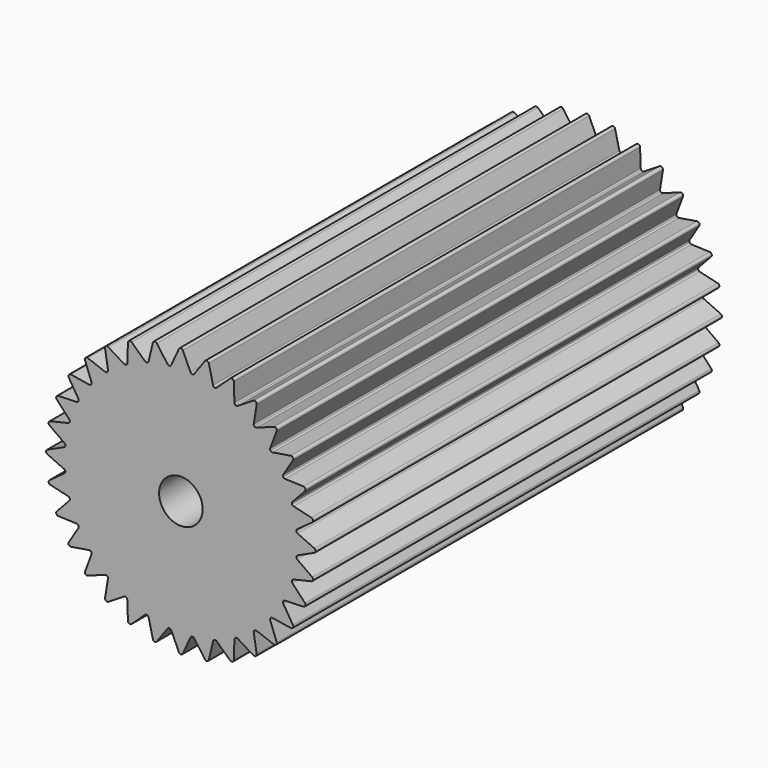
from build123d import *

# Parameters (mm, degrees)
F0_R            = 8
F0_R_2          = 5
F1_DEPTH        = 35
F2_DEPTH        = 20
F5_DEPTH        = 35
F5_COPIES_COUNT = 32
F6_T1_DEPTH     = 35
F6_T3_DEPTH     = 36.6415271023
F7_R            = 1.5
F8_DEPTH        = 8
F9_R            = 6
F10_DEPTH       = 25


# Not quite as in the source:
# - a fillet or chamfer that OpenCascade refuses, or shapes differently, is made with other operations: its cross-section is extruded or revolved along the edge and cut away or added
# - a pattern or mirror of a feature is missing from the dataset's text; its kind, count and spacing are read off the source's solid


with BuildPart() as f1:
    # F0 (on Front) → F1 (new body)
    with BuildSketch(Plane.XZ):
        Circle(F0_R)
        Circle(F0_R_2, mode=Mode.SUBTRACT)
        Circle(F0_R_2)
    extrude(amount=F1_DEPTH)

    # F0 (on Front) → F2 (join)
    with BuildSketch(Plane.XZ):
        Circle(F0_R_2)
    extrude(amount=F2_DEPTH)

    # F4 (on face) → F5 (join)
    with BuildSketch(Plane(origin=(0, 0, 0), x_dir=(-1, 0, 0), z_dir=(0, 1, 0))):
        with BuildLine():
            ThreePointArc((-0.6993297572, 7.969375), (-0.35, 7.9923400829), (0, 8))
            ThreePointArc((0, 8), (0.35, 7.9923400829), (0.6993297572, 7.969375))
            Line((0.6993297572, 7.969375), (0, 9.5))
            Line((0, 9.5), (-0.6993297572, 7.969375))
        make_face()
    f5 = extrude(amount=-F5_DEPTH)

    # F5_copies: F5 ×32 about axis
    f5_copies_axis = Axis((0, 0, 0), (0, 1, 0))
    for i in range(1, F5_COPIES_COUNT):
        add(f5.rotate(f5_copies_axis, i * 360 / F5_COPIES_COUNT))

    # F6: fillet of radius 0.15 on 96 edges, made by hand

    # F6_s2 → F6_t1 (join)
    with BuildSketch(Plane.XZ):
        with BuildLine():
            ThreePointArc((0.6632529517, 8.0483364054), (0.7125009612, 7.9886122754), (0.7849689133, 7.9613958453))
            ThreePointArc((0.7849689133, 7.9613958453), (0.7421600586, 7.9655005146), (0.6993297572, 7.969375))
            Line((0.6993297572, 7.969375), (0.6632529517, 8.0483364054))
        make_face()
        with BuildLine():
            ThreePointArc((-0.7849689133, 7.9613958453), (-0.7125009612, 7.9886122754), (-0.6632529517, 8.0483364054))
            Line((-0.6632529517, 8.0483364054), (-0.6993297572, 7.969375))
            ThreePointArc((-0.6993297572, 7.969375), (-0.7421600586, 7.9655005146), (-0.7849689133, 7.9613958453))
        make_face()
        with BuildLine():
            ThreePointArc((-0.7833053234, 7.9615596946), (-0.8596904862, 7.9741153725), (-0.9196438088, 8.0230841101))
            Line((-0.9196438088, 8.0230841101), (-0.868855603, 7.9526781616))
            ThreePointArc((-0.868855603, 7.9526781616), (-0.8260923992, 7.9572339005), (-0.7833053234, 7.9615596946))
        make_face()
        with BuildLine():
            ThreePointArc((-2.3214775758, 7.6557652697), (-2.3988445104, 7.6531776878), (-2.4671991735, 7.6895091918))
            Line((-2.4671991735, 7.6895091918), (-2.4036513296, 7.6303643613))
            ThreePointArc((-2.4036513296, 7.6303643613), (-2.3625985894, 7.6431752502), (-2.3214775758, 7.6557652697))
        make_face()
        with BuildLine():
            ThreePointArc((-2.3230772349, 7.6552800184), (-2.2573113963, 7.6961112886), (-2.2206612733, 7.7642956462))
            Line((-2.2206612733, 7.7642956462), (-2.2406402671, 7.6798132265))
            ThreePointArc((-2.2406402671, 7.6798132265), (-2.2818917216, 7.6676574109), (-2.3230772349, 7.6552800184))
        make_face()
        with BuildLine():
            ThreePointArc((-3.6927308274, 7.1818773596), (-3.7153746204, 7.107853061), (-3.7719110012, 7.0549760736))
            ThreePointArc((-3.7719110012, 7.0549760736), (-3.7339315654, 7.075150533), (-3.695844228, 7.0951205375))
            Line((-3.695844228, 7.0951205375), (-3.6927308274, 7.1818773596))
        make_face()
        with BuildLine():
            ThreePointArc((-3.7704367469, 7.0557640789), (-3.8458122853, 7.0381326765), (-3.9199414575, 7.0604307476))
            Line((-3.9199414575, 7.0604307476), (-3.8460760836, 7.0148199377))
            ThreePointArc((-3.8460760836, 7.0148199377), (-3.8083114408, 7.0353936613), (-3.7704367469, 7.0557640789))
        make_face()
        with BuildLine():
            ThreePointArc((-5.0228908068, 6.3234635537), (-5.0306580813, 6.2464440264), (-5.0757923429, 6.1835533548))
            ThreePointArc((-5.0757923429, 6.1835533548), (-5.0424785132, 6.2107495879), (-5.0090189679, 6.2377663454))
            Line((-5.0090189679, 6.2377663454), (-5.0228908068, 6.3234635537))
        make_face()
        with BuildLine():
            ThreePointArc((-5.0745001483, 6.1846138315), (-5.1449876509, 6.1526161735), (-5.2220425897, 6.1600239093))
            Line((-5.2220425897, 6.1600239093), (-5.1406982907, 6.129699918))
            ThreePointArc((-5.1406982907, 6.129699918), (-5.1076730192, 6.1572458396), (-5.0745001483, 6.1846138315))
        make_face()
        with BuildLine():
            ThreePointArc((-6.1600239093, 5.2220425897), (-6.1526161735, 5.1449876509), (-6.1846138315, 5.0745001483))
            ThreePointArc((-6.1846138315, 5.0745001483), (-6.1572458396, 5.1076730192), (-6.129699918, 5.1406982907))
            Line((-6.129699918, 5.1406982907), (-6.1600239093, 5.2220425897))
        make_face()
        with BuildLine():
            ThreePointArc((-6.1835533548, 5.0757923429), (-6.2464440264, 5.0306580813), (-6.3234635537, 5.0228908068))
            Line((-6.3234635537, 5.0228908068), (-6.2377663454, 5.0090189679))
            ThreePointArc((-6.2377663454, 5.0090189679), (-6.2107495879, 5.0424785132), (-6.1835533548, 5.0757923429))
        make_face()
        with BuildLine():
            ThreePointArc((-7.0604307476, 3.9199414575), (-7.0381326765, 3.8458122853), (-7.0557640789, 3.7704367469))
            ThreePointArc((-7.0557640789, 3.7704367469), (-7.0353936613, 3.8083114408), (-7.0148199377, 3.8460760836))
            Line((-7.0148199377, 3.8460760836), (-7.0604307476, 3.9199414575))
        make_face()
        with BuildLine():
            ThreePointArc((-7.0549760736, 3.7719110012), (-7.107853061, 3.7153746204), (-7.1818773596, 3.6927308274))
            Line((-7.1818773596, 3.6927308274), (-7.0951205375, 3.695844228))
            ThreePointArc((-7.0951205375, 3.695844228), (-7.075150533, 3.7339315654), (-7.0549760736, 3.7719110012))
        make_face()
        with BuildLine():
            ThreePointArc((-7.6895091918, 2.4671991735), (-7.6531776878, 2.3988445104), (-7.6557652697, 2.3214775758))
            ThreePointArc((-7.6557652697, 2.3214775758), (-7.6431752502, 2.3625985894), (-7.6303643613, 2.4036513296))
            Line((-7.6303643613, 2.4036513296), (-7.6895091918, 2.4671991735))
        make_face()
        with BuildLine():
            ThreePointArc((-7.6552800184, 2.3230772349), (-7.6961112886, 2.2573113963), (-7.7642956462, 2.2206612733))
            Line((-7.7642956462, 2.2206612733), (-7.6798132265, 2.2406402671))
            ThreePointArc((-7.6798132265, 2.2406402671), (-7.6676574109, 2.2818917216), (-7.6552800184, 2.3230772349))
        make_face()
        with BuildLine():
            ThreePointArc((-8.0230841101, 0.9196438088), (-7.9741153725, 0.8596904862), (-7.9615596946, 0.7833053234))
            ThreePointArc((-7.9615596946, 0.7833053234), (-7.9572339005, 0.8260923992), (-7.9526781616, 0.868855603))
            Line((-7.9526781616, 0.868855603), (-8.0230841101, 0.9196438088))
        make_face()
        with BuildLine():
            ThreePointArc((-7.9613958453, 0.7849689133), (-7.9886122754, 0.7125009612), (-8.0483364054, 0.6632529517))
            Line((-8.0483364054, 0.6632529517), (-7.969375, 0.6993297572))
            ThreePointArc((-7.969375, 0.6993297572), (-7.9655005146, 0.7421600586), (-7.9613958453, 0.7849689133))
        make_face()
        with BuildLine():
            ThreePointArc((-8.0483364054, -0.6632529517), (-7.9886122754, -0.7125009612), (-7.9613958453, -0.7849689133))
            ThreePointArc((-7.9613958453, -0.7849689133), (-7.9655005146, -0.7421600586), (-7.969375, -0.6993297572))
            Line((-7.969375, -0.6993297572), (-8.0483364054, -0.6632529517))
        make_face()
        with BuildLine():
            ThreePointArc((-7.9615596946, -0.7833053234), (-7.9741153725, -0.8596904862), (-8.0230841101, -0.9196438088))
            Line((-8.0230841101, -0.9196438088), (-7.9526781616, -0.868855603))
            ThreePointArc((-7.9526781616, -0.868855603), (-7.9572339005, -0.8260923992), (-7.9615596946, -0.7833053234))
        make_face()
        with BuildLine():
            ThreePointArc((-7.7642956462, -2.2206612733), (-7.6961112886, -2.2573113963), (-7.6552800184, -2.3230772349))
            ThreePointArc((-7.6552800184, -2.3230772349), (-7.6676574109, -2.2818917216), (-7.6798132265, -2.2406402671))
            Line((-7.6798132265, -2.2406402671), (-7.7642956462, -2.2206612733))
        make_face()
        with BuildLine():
            ThreePointArc((-7.6557652697, -2.3214775758), (-7.6531776878, -2.3988445104), (-7.6895091918, -2.4671991735))
            Line((-7.6895091918, -2.4671991735), (-7.6303643613, -2.4036513296))
            ThreePointArc((-7.6303643613, -2.4036513296), (-7.6431752502, -2.3625985894), (-7.6557652697, -2.3214775758))
        make_face()
        with BuildLine():
            ThreePointArc((-7.1818773596, -3.6927308274), (-7.107853061, -3.7153746204), (-7.0549760736, -3.7719110012))
            ThreePointArc((-7.0549760736, -3.7719110012), (-7.075150533, -3.7339315654), (-7.0951205375, -3.695844228))
            Line((-7.0951205375, -3.695844228), (-7.1818773596, -3.6927308274))
        make_face()
        with BuildLine():
            ThreePointArc((-7.0557640789, -3.7704367469), (-7.0381326765, -3.8458122853), (-7.0604307476, -3.9199414575))
            Line((-7.0604307476, -3.9199414575), (-7.0148199377, -3.8460760836))
            ThreePointArc((-7.0148199377, -3.8460760836), (-7.0353936613, -3.8083114408), (-7.0557640789, -3.7704367469))
        make_face()
        with BuildLine():
            ThreePointArc((-6.3234635537, -5.0228908068), (-6.2464440264, -5.0306580813), (-6.1835533548, -5.0757923429))
            ThreePointArc((-6.1835533548, -5.0757923429), (-6.2107495879, -5.0424785132), (-6.2377663454, -5.0090189679))
            Line((-6.2377663454, -5.0090189679), (-6.3234635537, -5.0228908068))
        make_face()
        with BuildLine():
            ThreePointArc((-6.1846138315, -5.0745001483), (-6.1526161735, -5.1449876509), (-6.1600239093, -5.2220425897))
            Line((-6.1600239093, -5.2220425897), (-6.129699918, -5.1406982907))
            ThreePointArc((-6.129699918, -5.1406982907), (-6.1572458396, -5.1076730192), (-6.1846138315, -5.0745001483))
        make_face()
        with BuildLine():
            ThreePointArc((-5.2220425897, -6.1600239093), (-5.1449876509, -6.1526161735), (-5.0745001483, -6.1846138315))
            ThreePointArc((-5.0745001483, -6.1846138315), (-5.1076730192, -6.1572458396), (-5.1406982907, -6.129699918))
            Line((-5.1406982907, -6.129699918), (-5.2220425897, -6.1600239093))
        make_face()
        with BuildLine():
            ThreePointArc((-5.0757923429, -6.1835533548), (-5.0306580813, -6.2464440264), (-5.0228908068, -6.3234635537))
            Line((-5.0228908068, -6.3234635537), (-5.0090189679, -6.2377663454))
            ThreePointArc((-5.0090189679, -6.2377663454), (-5.0424785132, -6.2107495879), (-5.0757923429, -6.1835533548))
        make_face()
        with BuildLine():
            ThreePointArc((-3.9199414575, -7.0604307476), (-3.8458122853, -7.0381326765), (-3.7704367469, -7.0557640789))
            ThreePointArc((-3.7704367469, -7.0557640789), (-3.8083114408, -7.0353936613), (-3.8460760836, -7.0148199377))
            Line((-3.8460760836, -7.0148199377), (-3.9199414575, -7.0604307476))
        make_face()
        with BuildLine():
            ThreePointArc((-3.7719110012, -7.0549760736), (-3.7153746204, -7.107853061), (-3.6927308274, -7.1818773596))
            Line((-3.6927308274, -7.1818773596), (-3.695844228, -7.0951205375))
            ThreePointArc((-3.695844228, -7.0951205375), (-3.7339315654, -7.075150533), (-3.7719110012, -7.0549760736))
        make_face()
        with BuildLine():
            ThreePointArc((-2.4671991735, -7.6895091918), (-2.3988445104, -7.6531776878), (-2.3214775758, -7.6557652697))
            ThreePointArc((-2.3214775758, -7.6557652697), (-2.3625985894, -7.6431752502), (-2.4036513296, -7.6303643613))
            Line((-2.4036513296, -7.6303643613), (-2.4671991735, -7.6895091918))
        make_face()
        with BuildLine():
            ThreePointArc((-2.3230772349, -7.6552800184), (-2.2573113963, -7.6961112886), (-2.2206612733, -7.7642956462))
            Line((-2.2206612733, -7.7642956462), (-2.2406402671, -7.6798132265))
            ThreePointArc((-2.2406402671, -7.6798132265), (-2.2818917216, -7.6676574109), (-2.3230772349, -7.6552800184))
        make_face()
        with BuildLine():
            ThreePointArc((-0.9196438088, -8.0230841101), (-0.8596904862, -7.9741153725), (-0.7833053234, -7.9615596946))
            ThreePointArc((-0.7833053234, -7.9615596946), (-0.8260923992, -7.9572339005), (-0.868855603, -7.9526781616))
            Line((-0.868855603, -7.9526781616), (-0.9196438088, -8.0230841101))
        make_face()
        with BuildLine():
            ThreePointArc((-0.7849689133, -7.9613958453), (-0.7125009612, -7.9886122754), (-0.6632529517, -8.0483364054))
            Line((-0.6632529517, -8.0483364054), (-0.6993297572, -7.969375))
            ThreePointArc((-0.6993297572, -7.969375), (-0.7421600586, -7.9655005146), (-0.7849689133, -7.9613958453))
        make_face()
        with BuildLine():
            ThreePointArc((0.6632529517, -8.0483364054), (0.7125009612, -7.9886122754), (0.7849689133, -7.9613958453))
            ThreePointArc((0.7849689133, -7.9613958453), (0.7421600586, -7.9655005146), (0.6993297572, -7.969375))
            Line((0.6993297572, -7.969375), (0.6632529517, -8.0483364054))
        make_face()
        with BuildLine():
            ThreePointArc((0.7833053234, -7.9615596946), (0.8596904862, -7.9741153725), (0.9196438088, -8.0230841101))
            Line((0.9196438088, -8.0230841101), (0.868855603, -7.9526781616))
            ThreePointArc((0.868855603, -7.9526781616), (0.8260923992, -7.9572339005), (0.7833053234, -7.9615596946))
        make_face()
        with BuildLine():
            ThreePointArc((2.2206612733, -7.7642956462), (2.2573113963, -7.6961112886), (2.3230772349, -7.6552800184))
            ThreePointArc((2.3230772349, -7.6552800184), (2.2818917216, -7.6676574109), (2.2406402671, -7.6798132265))
            Line((2.2406402671, -7.6798132265), (2.2206612733, -7.7642956462))
        make_face()
        with BuildLine():
            ThreePointArc((2.3214775758, -7.6557652697), (2.3988445104, -7.6531776878), (2.4671991735, -7.6895091918))
            Line((2.4671991735, -7.6895091918), (2.4036513296, -7.6303643613))
            ThreePointArc((2.4036513296, -7.6303643613), (2.3625985894, -7.6431752502), (2.3214775758, -7.6557652697))
        make_face()
        with BuildLine():
            ThreePointArc((3.6927308274, -7.1818773596), (3.7153746204, -7.107853061), (3.7719110012, -7.0549760736))
            ThreePointArc((3.7719110012, -7.0549760736), (3.7339315654, -7.075150533), (3.695844228, -7.0951205375))
            Line((3.695844228, -7.0951205375), (3.6927308274, -7.1818773596))
        make_face()
        with BuildLine():
            ThreePointArc((3.7704367469, -7.0557640789), (3.8458122853, -7.0381326765), (3.9199414575, -7.0604307476))
            Line((3.9199414575, -7.0604307476), (3.8460760836, -7.0148199377))
            ThreePointArc((3.8460760836, -7.0148199377), (3.8083114408, -7.0353936613), (3.7704367469, -7.0557640789))
        make_face()
        with BuildLine():
            ThreePointArc((5.0228908068, -6.3234635537), (5.0306580813, -6.2464440264), (5.0757923429, -6.1835533548))
            ThreePointArc((5.0757923429, -6.1835533548), (5.0424785132, -6.2107495879), (5.0090189679, -6.2377663454))
            Line((5.0090189679, -6.2377663454), (5.0228908068, -6.3234635537))
        make_face()
        with BuildLine():
            ThreePointArc((5.0745001483, -6.1846138315), (5.1449876509, -6.1526161735), (5.2220425897, -6.1600239093))
            Line((5.2220425897, -6.1600239093), (5.1406982907, -6.129699918))
            ThreePointArc((5.1406982907, -6.129699918), (5.1076730192, -6.1572458396), (5.0745001483, -6.1846138315))
        make_face()
        with BuildLine():
            ThreePointArc((6.1600239093, -5.2220425897), (6.1526161735, -5.1449876509), (6.1846138315, -5.0745001483))
            ThreePointArc((6.1846138315, -5.0745001483), (6.1572458396, -5.1076730192), (6.129699918, -5.1406982907))
            Line((6.129699918, -5.1406982907), (6.1600239093, -5.2220425897))
        make_face()
        with BuildLine():
            ThreePointArc((6.1835533548, -5.0757923429), (6.2464440264, -5.0306580813), (6.3234635537, -5.0228908068))
            Line((6.3234635537, -5.0228908068), (6.2377663454, -5.0090189679))
            ThreePointArc((6.2377663454, -5.0090189679), (6.2107495879, -5.0424785132), (6.1835533548, -5.0757923429))
        make_face()
        with BuildLine():
            ThreePointArc((7.0604307476, -3.9199414575), (7.0381326765, -3.8458122853), (7.0557640789, -3.7704367469))
            ThreePointArc((7.0557640789, -3.7704367469), (7.0353936613, -3.8083114408), (7.0148199377, -3.8460760836))
            Line((7.0148199377, -3.8460760836), (7.0604307476, -3.9199414575))
        make_face()
        with BuildLine():
            ThreePointArc((7.0549760736, -3.7719110012), (7.107853061, -3.7153746204), (7.1818773596, -3.6927308274))
            Line((7.1818773596, -3.6927308274), (7.0951205375, -3.695844228))
            ThreePointArc((7.0951205375, -3.695844228), (7.075150533, -3.7339315654), (7.0549760736, -3.7719110012))
        make_face()
        with BuildLine():
            ThreePointArc((7.6895091918, -2.4671991735), (7.6531776878, -2.3988445104), (7.6557652697, -2.3214775758))
            ThreePointArc((7.6557652697, -2.3214775758), (7.6431752502, -2.3625985894), (7.6303643613, -2.4036513296))
            Line((7.6303643613, -2.4036513296), (7.6895091918, -2.4671991735))
        make_face()
        with BuildLine():
            ThreePointArc((7.6552800184, -2.3230772349), (7.6961112886, -2.2573113963), (7.7642956462, -2.2206612733))
            Line((7.7642956462, -2.2206612733), (7.6798132265, -2.2406402671))
            ThreePointArc((7.6798132265, -2.2406402671), (7.6676574109, -2.2818917216), (7.6552800184, -2.3230772349))
        make_face()
        with BuildLine():
            ThreePointArc((8.0230841101, -0.9196438088), (7.9741153725, -0.8596904862), (7.9615596946, -0.7833053234))
            ThreePointArc((7.9615596946, -0.7833053234), (7.9572339005, -0.8260923992), (7.9526781616, -0.868855603))
            Line((7.9526781616, -0.868855603), (8.0230841101, -0.9196438088))
        make_face()
        with BuildLine():
            ThreePointArc((7.9613958453, -0.7849689133), (7.9886122754, -0.7125009612), (8.0483364054, -0.6632529517))
            Line((8.0483364054, -0.6632529517), (7.969375, -0.6993297572))
            ThreePointArc((7.969375, -0.6993297572), (7.9655005146, -0.7421600586), (7.9613958453, -0.7849689133))
        make_face()
        with BuildLine():
            ThreePointArc((8.0483364054, 0.6632529517), (7.9886122754, 0.7125009612), (7.9613958453, 0.7849689133))
            ThreePointArc((7.9613958453, 0.7849689133), (7.9655005146, 0.7421600586), (7.969375, 0.6993297572))
            Line((7.969375, 0.6993297572), (8.0483364054, 0.6632529517))
        make_face()
        with BuildLine():
            ThreePointArc((7.9615596946, 0.7833053234), (7.9741153725, 0.8596904862), (8.0230841101, 0.9196438088))
            Line((8.0230841101, 0.9196438088), (7.9526781616, 0.868855603))
            ThreePointArc((7.9526781616, 0.868855603), (7.9572339005, 0.8260923992), (7.9615596946, 0.7833053234))
        make_face()
        with BuildLine():
            ThreePointArc((7.7642956462, 2.2206612733), (7.6961112886, 2.2573113963), (7.6552800184, 2.3230772349))
            ThreePointArc((7.6552800184, 2.3230772349), (7.6676574109, 2.2818917216), (7.6798132265, 2.2406402671))
            Line((7.6798132265, 2.2406402671), (7.7642956462, 2.2206612733))
        make_face()
        with BuildLine():
            ThreePointArc((7.6557652697, 2.3214775758), (7.6531776878, 2.3988445104), (7.6895091918, 2.4671991735))
            Line((7.6895091918, 2.4671991735), (7.6303643613, 2.4036513296))
            ThreePointArc((7.6303643613, 2.4036513296), (7.6431752502, 2.3625985894), (7.6557652697, 2.3214775758))
        make_face()
        with BuildLine():
            ThreePointArc((7.1818773596, 3.6927308274), (7.107853061, 3.7153746204), (7.0549760736, 3.7719110012))
            ThreePointArc((7.0549760736, 3.7719110012), (7.075150533, 3.7339315654), (7.0951205375, 3.695844228))
            Line((7.0951205375, 3.695844228), (7.1818773596, 3.6927308274))
        make_face()
        with BuildLine():
            ThreePointArc((7.0557640789, 3.7704367469), (7.0381326765, 3.8458122853), (7.0604307476, 3.9199414575))
            Line((7.0604307476, 3.9199414575), (7.0148199377, 3.8460760836))
            ThreePointArc((7.0148199377, 3.8460760836), (7.0353936613, 3.8083114408), (7.0557640789, 3.7704367469))
        make_face()
        with BuildLine():
            ThreePointArc((6.3234635537, 5.0228908068), (6.2464440264, 5.0306580813), (6.1835533548, 5.0757923429))
            ThreePointArc((6.1835533548, 5.0757923429), (6.2107495879, 5.0424785132), (6.2377663454, 5.0090189679))
            Line((6.2377663454, 5.0090189679), (6.3234635537, 5.0228908068))
        make_face()
        with BuildLine():
            ThreePointArc((6.1846138315, 5.0745001483), (6.1526161735, 5.1449876509), (6.1600239093, 5.2220425897))
            Line((6.1600239093, 5.2220425897), (6.129699918, 5.1406982907))
            ThreePointArc((6.129699918, 5.1406982907), (6.1572458396, 5.1076730192), (6.1846138315, 5.0745001483))
        make_face()
        with BuildLine():
            ThreePointArc((5.2220425897, 6.1600239093), (5.1449876509, 6.1526161735), (5.0745001483, 6.1846138315))
            ThreePointArc((5.0745001483, 6.1846138315), (5.1076730192, 6.1572458396), (5.1406982907, 6.129699918))
            Line((5.1406982907, 6.129699918), (5.2220425897, 6.1600239093))
        make_face()
        with BuildLine():
            ThreePointArc((5.0757923429, 6.1835533548), (5.0306580813, 6.2464440264), (5.0228908068, 6.3234635537))
            Line((5.0228908068, 6.3234635537), (5.0090189679, 6.2377663454))
            ThreePointArc((5.0090189679, 6.2377663454), (5.0424785132, 6.2107495879), (5.0757923429, 6.1835533548))
        make_face()
        with BuildLine():
            ThreePointArc((3.9199414575, 7.0604307476), (3.8458122853, 7.0381326765), (3.7704367469, 7.0557640789))
            ThreePointArc((3.7704367469, 7.0557640789), (3.8083114408, 7.0353936613), (3.8460760836, 7.0148199377))
            Line((3.8460760836, 7.0148199377), (3.9199414575, 7.0604307476))
        make_face()
        with BuildLine():
            ThreePointArc((3.7719110012, 7.0549760736), (3.7153746204, 7.107853061), (3.6927308274, 7.1818773596))
            Line((3.6927308274, 7.1818773596), (3.695844228, 7.0951205375))
            ThreePointArc((3.695844228, 7.0951205375), (3.7339315654, 7.075150533), (3.7719110012, 7.0549760736))
        make_face()
        with BuildLine():
            ThreePointArc((2.4671991735, 7.6895091918), (2.3988445104, 7.6531776878), (2.3214775758, 7.6557652697))
            ThreePointArc((2.3214775758, 7.6557652697), (2.3625985894, 7.6431752502), (2.4036513296, 7.6303643613))
            Line((2.4036513296, 7.6303643613), (2.4671991735, 7.6895091918))
        make_face()
        with BuildLine():
            ThreePointArc((2.3230772349, 7.6552800184), (2.2573113963, 7.6961112886), (2.2206612733, 7.7642956462))
            Line((2.2206612733, 7.7642956462), (2.2406402671, 7.6798132265))
            ThreePointArc((2.2406402671, 7.6798132265), (2.2818917216, 7.6676574109), (2.3230772349, 7.6552800184))
        make_face()
        with BuildLine():
            ThreePointArc((0.9196438088, 8.0230841101), (0.8596904862, 7.9741153725), (0.7833053234, 7.9615596946))
            ThreePointArc((0.7833053234, 7.9615596946), (0.8260923992, 7.9572339005), (0.868855603, 7.9526781616))
            Line((0.868855603, 7.9526781616), (0.9196438088, 8.0230841101))
        make_face()
    extrude(amount=F6_T1_DEPTH)

    # F6_s4 → F6_t3 (cut)
    with BuildSketch(Plane.XZ.offset(-0.8207635512)):
        with BuildLine():
            ThreePointArc((0.1364341287, 9.20138624), (0, 9.2890506281), (-0.1364341287, 9.20138624))
            Line((-0.1364341287, 9.20138624), (0, 9.5))
            Line((0, 9.5), (0.1364341287, 9.20138624))
        make_face()
        with BuildLine():
            ThreePointArc((-1.6612888194, 9.0512011616), (-1.8122038783, 9.1105641249), (-1.9289139898, 8.9979672054))
            Line((-1.9289139898, 8.9979672054), (-1.8533580592, 9.3174601638))
            Line((-1.8533580592, 9.3174601638), (-1.6612888194, 9.0512011616))
        make_face()
        with BuildLine():
            ThreePointArc((-3.3951693698, 8.5531834986), (-3.5547657778, 8.5819637517), (-3.6472667679, 8.4487613372))
            Line((-3.6472667679, 8.4487613372), (-3.6354926075, 8.7768555589))
            Line((-3.6354926075, 8.7768555589), (-3.3951693698, 8.5531834986))
        make_face()
        with BuildLine():
            ThreePointArc((-4.9985754654, 7.7264717903), (-5.160720022, 7.7235633244), (-5.2254571296, 7.574874309))
            Line((-5.2254571296, 7.574874309), (-5.2779172137, 7.8989613169))
            Line((-5.2779172137, 7.8989613169), (-4.9985754654, 7.7264717903))
        make_face()
        with BuildLine():
            ThreePointArc((-6.4098891091, 6.6028361043), (-6.5683506899, 6.5683506899), (-6.6028361043, 6.4098891091))
            Line((-6.6028361043, 6.4098891091), (-6.7175144213, 6.7175144213))
            Line((-6.7175144213, 6.7175144213), (-6.4098891091, 6.6028361043))
        make_face()
        with BuildLine():
            ThreePointArc((-7.574874309, 5.2254571296), (-7.7235633244, 5.160720022), (-7.7264717903, 4.9985754654))
            Line((-7.7264717903, 4.9985754654), (-7.8989613169, 5.2779172137))
            Line((-7.8989613169, 5.2779172137), (-7.574874309, 5.2254571296))
        make_face()
        with BuildLine():
            ThreePointArc((-8.4487613372, 3.6472667679), (-8.5819637517, 3.5547657778), (-8.5531834986, 3.3951693698))
            Line((-8.5531834986, 3.3951693698), (-8.7768555589, 3.6354926075))
            Line((-8.7768555589, 3.6354926075), (-8.4487613372, 3.6472667679))
        make_face()
        with BuildLine():
            ThreePointArc((-8.9979672054, 1.9289139898), (-9.1105641249, 1.8122038783), (-9.0512011616, 1.6612888194))
            Line((-9.0512011616, 1.6612888194), (-9.3174601638, 1.8533580592))
            Line((-9.3174601638, 1.8533580592), (-8.9979672054, 1.9289139898))
        make_face()
        with BuildLine():
            ThreePointArc((-9.20138624, 0.1364341287), (-9.2890506281, 0), (-9.20138624, -0.1364341287))
            Line((-9.20138624, -0.1364341287), (-9.5, 0))
            Line((-9.5, 0), (-9.20138624, 0.1364341287))
        make_face()
        with BuildLine():
            ThreePointArc((-9.0512011616, -1.6612888194), (-9.1105641249, -1.8122038783), (-8.9979672054, -1.9289139898))
            Line((-8.9979672054, -1.9289139898), (-9.3174601638, -1.8533580592))
            Line((-9.3174601638, -1.8533580592), (-9.0512011616, -1.6612888194))
        make_face()
        with BuildLine():
            ThreePointArc((-8.5531834986, -3.3951693698), (-8.5819637517, -3.5547657778), (-8.4487613372, -3.6472667679))
            Line((-8.4487613372, -3.6472667679), (-8.7768555589, -3.6354926075))
            Line((-8.7768555589, -3.6354926075), (-8.5531834986, -3.3951693698))
        make_face()
        with BuildLine():
            ThreePointArc((-7.7264717903, -4.9985754654), (-7.7235633244, -5.160720022), (-7.574874309, -5.2254571296))
            Line((-7.574874309, -5.2254571296), (-7.8989613169, -5.2779172137))
            Line((-7.8989613169, -5.2779172137), (-7.7264717903, -4.9985754654))
        make_face()
        with BuildLine():
            ThreePointArc((-6.6028361043, -6.4098891091), (-6.5683506899, -6.5683506899), (-6.4098891091, -6.6028361043))
            Line((-6.4098891091, -6.6028361043), (-6.7175144213, -6.7175144213))
            Line((-6.7175144213, -6.7175144213), (-6.6028361043, -6.4098891091))
        make_face()
        with BuildLine():
            ThreePointArc((-5.2254571296, -7.574874309), (-5.160720022, -7.7235633244), (-4.9985754654, -7.7264717903))
            Line((-4.9985754654, -7.7264717903), (-5.2779172137, -7.8989613169))
            Line((-5.2779172137, -7.8989613169), (-5.2254571296, -7.574874309))
        make_face()
        with BuildLine():
            ThreePointArc((-3.6472667679, -8.4487613372), (-3.5547657778, -8.5819637517), (-3.3951693698, -8.5531834986))
            Line((-3.3951693698, -8.5531834986), (-3.6354926075, -8.7768555589))
            Line((-3.6354926075, -8.7768555589), (-3.6472667679, -8.4487613372))
        make_face()
        with BuildLine():
            ThreePointArc((-1.9289139898, -8.9979672054), (-1.8122038783, -9.1105641249), (-1.6612888194, -9.0512011616))
            Line((-1.6612888194, -9.0512011616), (-1.8533580592, -9.3174601638))
            Line((-1.8533580592, -9.3174601638), (-1.9289139898, -8.9979672054))
        make_face()
        with BuildLine():
            ThreePointArc((-0.1364341287, -9.20138624), (0, -9.2890506281), (0.1364341287, -9.20138624))
            Line((0.1364341287, -9.20138624), (0, -9.5))
            Line((0, -9.5), (-0.1364341287, -9.20138624))
        make_face()
        with BuildLine():
            ThreePointArc((1.6612888194, -9.0512011616), (1.8122038783, -9.1105641249), (1.9289139898, -8.9979672054))
            Line((1.9289139898, -8.9979672054), (1.8533580592, -9.3174601638))
            Line((1.8533580592, -9.3174601638), (1.6612888194, -9.0512011616))
        make_face()
        with BuildLine():
            ThreePointArc((3.3951693698, -8.5531834986), (3.5547657778, -8.5819637517), (3.6472667679, -8.4487613372))
            Line((3.6472667679, -8.4487613372), (3.6354926075, -8.7768555589))
            Line((3.6354926075, -8.7768555589), (3.3951693698, -8.5531834986))
        make_face()
        with BuildLine():
            ThreePointArc((4.9985754654, -7.7264717903), (5.160720022, -7.7235633244), (5.2254571296, -7.574874309))
            Line((5.2254571296, -7.574874309), (5.2779172137, -7.8989613169))
            Line((5.2779172137, -7.8989613169), (4.9985754654, -7.7264717903))
        make_face()
        with BuildLine():
            ThreePointArc((6.4098891091, -6.6028361043), (6.5683506899, -6.5683506899), (6.6028361043, -6.4098891091))
            Line((6.6028361043, -6.4098891091), (6.7175144213, -6.7175144213))
            Line((6.7175144213, -6.7175144213), (6.4098891091, -6.6028361043))
        make_face()
        with BuildLine():
            ThreePointArc((7.574874309, -5.2254571296), (7.7235633244, -5.160720022), (7.7264717903, -4.9985754654))
            Line((7.7264717903, -4.9985754654), (7.8989613169, -5.2779172137))
            Line((7.8989613169, -5.2779172137), (7.574874309, -5.2254571296))
        make_face()
        with BuildLine():
            ThreePointArc((8.4487613372, -3.6472667679), (8.5819637517, -3.5547657778), (8.5531834986, -3.3951693698))
            Line((8.5531834986, -3.3951693698), (8.7768555589, -3.6354926075))
            Line((8.7768555589, -3.6354926075), (8.4487613372, -3.6472667679))
        make_face()
        with BuildLine():
            ThreePointArc((8.9979672054, -1.9289139898), (9.1105641249, -1.8122038783), (9.0512011616, -1.6612888194))
            Line((9.0512011616, -1.6612888194), (9.3174601638, -1.8533580592))
            Line((9.3174601638, -1.8533580592), (8.9979672054, -1.9289139898))
        make_face()
        with BuildLine():
            ThreePointArc((9.20138624, -0.1364341287), (9.2890506281, 0), (9.20138624, 0.1364341287))
            Line((9.20138624, 0.1364341287), (9.5, 0))
            Line((9.5, 0), (9.20138624, -0.1364341287))
        make_face()
        with BuildLine():
            ThreePointArc((9.0512011616, 1.6612888194), (9.1105641249, 1.8122038783), (8.9979672054, 1.9289139898))
            Line((8.9979672054, 1.9289139898), (9.3174601638, 1.8533580592))
            Line((9.3174601638, 1.8533580592), (9.0512011616, 1.6612888194))
        make_face()
        with BuildLine():
            ThreePointArc((8.5531834986, 3.3951693698), (8.5819637517, 3.5547657778), (8.4487613372, 3.6472667679))
            Line((8.4487613372, 3.6472667679), (8.7768555589, 3.6354926075))
            Line((8.7768555589, 3.6354926075), (8.5531834986, 3.3951693698))
        make_face()
        with BuildLine():
            ThreePointArc((7.7264717903, 4.9985754654), (7.7235633244, 5.160720022), (7.574874309, 5.2254571296))
            Line((7.574874309, 5.2254571296), (7.8989613169, 5.2779172137))
            Line((7.8989613169, 5.2779172137), (7.7264717903, 4.9985754654))
        make_face()
        with BuildLine():
            ThreePointArc((6.6028361043, 6.4098891091), (6.5683506899, 6.5683506899), (6.4098891091, 6.6028361043))
            Line((6.4098891091, 6.6028361043), (6.7175144213, 6.7175144213))
            Line((6.7175144213, 6.7175144213), (6.6028361043, 6.4098891091))
        make_face()
        with BuildLine():
            ThreePointArc((5.2254571296, 7.574874309), (5.160720022, 7.7235633244), (4.9985754654, 7.7264717903))
            Line((4.9985754654, 7.7264717903), (5.2779172137, 7.8989613169))
            Line((5.2779172137, 7.8989613169), (5.2254571296, 7.574874309))
        make_face()
        with BuildLine():
            ThreePointArc((3.6472667679, 8.4487613372), (3.5547657778, 8.5819637517), (3.3951693698, 8.5531834986))
            Line((3.3951693698, 8.5531834986), (3.6354926075, 8.7768555589))
            Line((3.6354926075, 8.7768555589), (3.6472667679, 8.4487613372))
        make_face()
        with BuildLine():
            ThreePointArc((1.9289139898, 8.9979672054), (1.8122038783, 9.1105641249), (1.6612888194, 9.0512011616))
            Line((1.6612888194, 9.0512011616), (1.8533580592, 9.3174601638))
            Line((1.8533580592, 9.3174601638), (1.9289139898, 8.9979672054))
        make_face()
    extrude(amount=F6_T3_DEPTH, mode=Mode.SUBTRACT)

    # F7 (on face) → F8 (cut)
    with BuildSketch(Plane.XZ.offset(35)):
        Circle(F7_R)
    extrude(amount=-F8_DEPTH, mode=Mode.SUBTRACT)

    # F9 (on face) → F10 (cut)
    with BuildSketch(Plane(origin=(0, 0, 0), x_dir=(-1, 0, 0), z_dir=(0, 1, 0))):
        Circle(F9_R)
    extrude(amount=-F10_DEPTH, mode=Mode.SUBTRACT)


solid = f1.part
